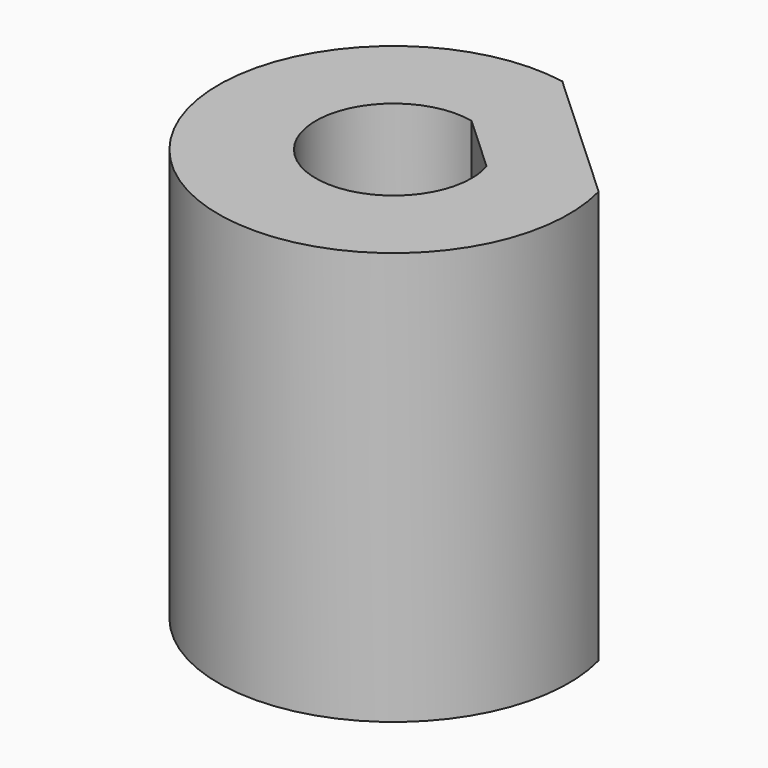
from build123d import *

# Parameters (mm, degrees)
F1_DEPTH = 35
F2_R     = 6.604
F3_DEPTH = 38.1
F5_DEPTH = 31.75


# Not quite as in the source:
# - a feature names something its author has since deleted; it is built from what else it names


with BuildPart() as f1:
    # F0 (on Top) → F1 (new body)
    with BuildSketch(Plane.XY):
        with BuildLine():
            Line((14.3630077291, 3.7718044718), (2.6000410284, 14.6206117058))
            ThreePointArc((2.6000410284, 14.6206117058), (-10.0677907401, -10.9161389517), (14.3630077291, 3.7718044718))
        make_face()
    extrude(amount=F1_DEPTH)

    # F2 (on face) → F3 (cut)
    with BuildSketch(Plane.XY.offset(35)):
        Circle(F2_R)
    extrude(amount=-F3_DEPTH, mode=Mode.SUBTRACT)

    # F4 (on face) → F5 (join)
    with BuildSketch(Plane.XY.offset(35)):
        with BuildLine():
            ThreePointArc((6.3047218477, 1.9655275177), (4.4772855251, 4.854557686), (1.4501641617, 6.4428130428))
            Line((1.4501641617, 6.4428130428), (6.3047218477, 1.9655275177))
        make_face()
    extrude(amount=-F5_DEPTH)


solid = f1.part
